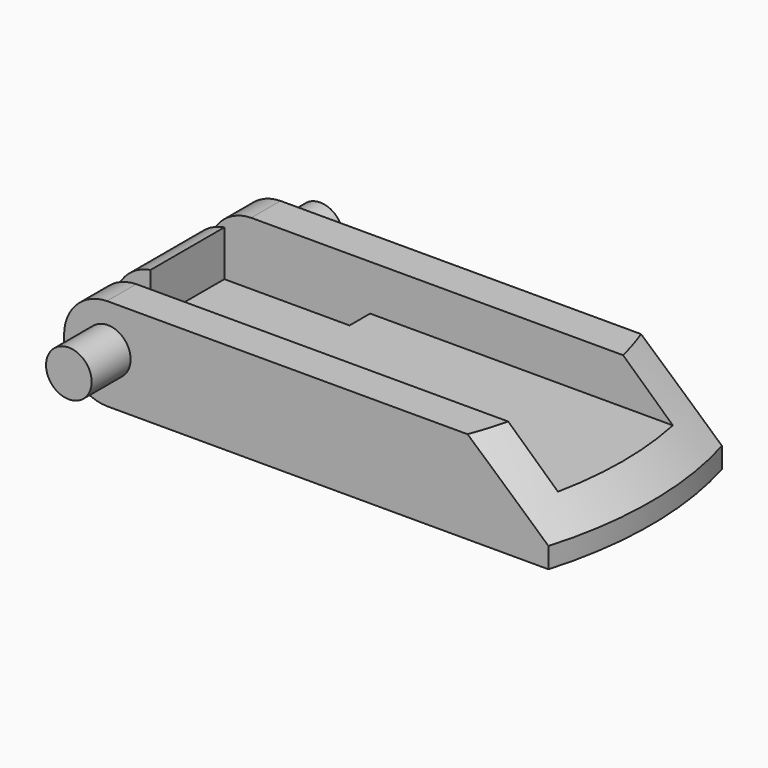
from build123d import *

# Parameters (mm, degrees)
F1_DEPTH     = 2.45
F2_W         = 1.91
F2_H         = 1.91
F2_H_2       = 4.81
F3_DEPTH     = 2.38
F4_T1_DEPTH  = 13.3148286025
F4_T3_DEPTH  = 7.6124143012
F4_T5_DEPTH  = 13.3148286025
F4_T7_DEPTH  = 16.0629874681
F4_T9_DEPTH  = 16.2148286025
F4_T14_DEPTH = 13.3148286025
F5_T2_ANGLE  = 64.9142912697
F5_T4_ANGLE  = 64.9142912697
F6_R         = 1.19
F7_DEPTH     = 2.54


# Not quite as in the source:
# - a fillet or chamfer that OpenCascade refuses, or shapes differently, is made with other operations: its cross-section is extruded or revolved along the edge and cut away or added


with BuildPart() as f1:
    # F0 (on Top) → F1 (new body)
    with BuildSketch(Plane.XY):
        Polygon((12.22, -5.655), (12.22, 5.655), (-7.02, 5.655), (-9.51, 5.655), (-13.04, 5.655), (-13.04, 3.745), (-4.6004378237, 3.745), (-4.6004378237, 2.405), (-13.04, 2.405), (-13.04, -2.405), (-4.6004378237, -2.405), (-4.6004378237, -3.745), (-13.04, -3.745), (-13.04, -5.655), (-9.51, -5.655), (-7.02, -5.655), align=None)
        with BuildLine():
            ThreePointArc((12.22, -5.655), (13.04, 0), (12.22, 5.655))
            Line((12.22, 5.655), (12.22, -5.655))
        make_face()
    extrude(amount=F1_DEPTH)

    # F2 (on face) → F3 (join)
    with BuildSketch(Plane.XY.offset(2.45)):
        with BuildLine():
            ThreePointArc((12.6846069362, 3.745), (12.4758901154, 4.705737445), (12.22, 5.655))
            Line((12.22, 5.655), (-11.13, 5.655))
            Line((-11.13, 5.655), (-11.13, 3.745))
            Line((-11.13, 3.745), (-4.6004378237, 3.745))
            Line((-4.6004378237, 3.745), (12.6846069362, 3.745))
        make_face()
        with Locations((-12.085, 4.7)):
            Rectangle(F2_W, F2_H)
        with Locations((-12.085, 0)):
            Rectangle(F2_W, F2_H_2)
        with Locations((-12.085, -4.7)):
            Rectangle(F2_W, F2_H)
        with BuildLine():
            ThreePointArc((12.22, -5.655), (12.4758901154, -4.705737445), (12.6846069362, -3.745))
            Line((12.6846069362, -3.745), (-4.6004378237, -3.745))
            Line((-4.6004378237, -3.745), (-11.13, -3.745))
            Line((-11.13, -3.745), (-11.13, -5.655))
            Line((-11.13, -5.655), (12.22, -5.655))
        make_face()
    extrude(amount=F3_DEPTH)

    # F4: fillet of radius 2.28 on 6 edges, made by hand

    # F4_s2 → F4_t1 (cut)
    with BuildSketch(Plane.XZ.offset(-1.9574143012)):
        with BuildLine():
            ThreePointArc((-10.7590343146, -0.0004), (-12.3722034611, 0.6677965389), (-13.0404, 2.2809656854))
            Line((-13.0404, 2.2809656854), (-13.2685365685, 2.2809656854))
            ThreePointArc((-13.2685365685, 2.2809656854), (-13.2681365685, 1.1404828427), (-13.2681365685, 0))
            Line((-13.2681365685, 0), (-13.04, -0.2281365685))
            ThreePointArc((-13.04, -0.2281365685), (-11.8995171573, -0.2281365685), (-10.7590343146, -0.2285365685))
            Line((-10.7590343146, -0.2285365685), (-10.7590343146, -0.0004))
        make_face()
    extrude(amount=F4_T1_DEPTH, mode=Mode.SUBTRACT)

    # F4_s4 → F4_t3 (cut)
    with BuildSketch(Plane.XZ.offset(-11.3574143012)):
        with BuildLine():
            ThreePointArc((-10.7590343146, 4.8304), (-12.3722034611, 4.1622034611), (-13.0404, 2.5490343146))
            Line((-13.0404, 2.5490343146), (-13.2685365685, 2.5490343146))
            ThreePointArc((-13.2685365685, 2.5490343146), (-13.2681365685, 3.6895171573), (-13.2681365685, 4.83))
            Line((-13.2681365685, 4.83), (-13.04, 5.0581365685))
            ThreePointArc((-13.04, 5.0581365685), (-11.8995171573, 5.0581365685), (-10.7590343146, 5.0585365685))
            Line((-10.7590343146, 5.0585365685), (-10.7590343146, 4.8304))
        make_face()
    extrude(amount=F4_T3_DEPTH, mode=Mode.SUBTRACT)

    # F4_s6 → F4_t5 (cut)
    with BuildSketch(Plane.XZ.offset(-11.3574143012)):
        with BuildLine():
            ThreePointArc((-10.7590343146, -0.0004), (-12.3722034611, 0.6677965389), (-13.0404, 2.2809656854))
            Line((-13.0404, 2.2809656854), (-13.2685365685, 2.2809656854))
            ThreePointArc((-13.2685365685, 2.2809656854), (-13.2681365685, 1.1404828427), (-13.2681365685, 0))
            Line((-13.2681365685, 0), (-13.04, -0.2281365685))
            ThreePointArc((-13.04, -0.2281365685), (-11.8995171573, -0.2281365685), (-10.7590343146, -0.2285365685))
            Line((-10.7590343146, -0.2285365685), (-10.7590343146, -0.0004))
        make_face()
    extrude(amount=F4_T5_DEPTH, mode=Mode.SUBTRACT)

    # F4_s8 → F4_t7 (cut)
    with BuildSketch(Plane.XZ.offset(-8.0314937341)):
        with BuildLine():
            ThreePointArc((-11.1300650541, 4.8303946745), (-12.4984431492, 4.0555753965), (-13.0404, 2.5794025419))
            Line((-13.0404, 2.5794025419), (-13.2685365685, 2.5794025419))
            ThreePointArc((-13.2685365685, 2.5794025419), (-13.2681365685, 3.704701271), (-13.2681365685, 4.83))
            Line((-13.2681365685, 4.83), (-13.04, 5.0581365685))
            ThreePointArc((-13.04, 5.0581365685), (-12.0850325271, 5.0581365685), (-11.1671681281, 5.0554938878))
            Line((-11.1671681281, 5.0554938878), (-11.1300650541, 4.8303946745))
        make_face()
    extrude(amount=F4_T7_DEPTH, mode=Mode.SUBTRACT)

    # F4_s10 → F4_t9 (cut)
    with BuildSketch(Plane.XZ.offset(-8.1074143012)):
        with BuildLine():
            ThreePointArc((-10.7590343146, -0.0004), (-12.3722034611, 0.6677965389), (-13.0404, 2.2809656854))
            Line((-13.0404, 2.2809656854), (-13.2685365685, 2.2809656854))
            ThreePointArc((-13.2685365685, 2.2809656854), (-13.2681365685, 1.1404828427), (-13.2681365685, 0))
            Line((-13.2681365685, 0), (-13.04, -0.2281365685))
            ThreePointArc((-13.04, -0.2281365685), (-11.8995171573, -0.2281365685), (-10.7590343146, -0.2285365685))
            Line((-10.7590343146, -0.2285365685), (-10.7590343146, -0.0004))
        make_face()
    extrude(amount=F4_T9_DEPTH, mode=Mode.SUBTRACT)


with BuildPart() as f4_tool12:
    # F4_s13 → F4_t14 (new body)
    with BuildSketch(Plane.XZ.offset(-1.9574143012)):
        with BuildLine():
            ThreePointArc((-10.7590343146, 4.8304), (-12.3722034611, 4.1622034611), (-13.0404, 2.5490343146))
            Line((-13.0404, 2.5490343146), (-13.2685365685, 2.5490343146))
            ThreePointArc((-13.2685365685, 2.5490343146), (-13.2681365685, 3.6895171573), (-13.2681365685, 4.83))
            Line((-13.2681365685, 4.83), (-13.04, 5.0581365685))
            ThreePointArc((-13.04, 5.0581365685), (-11.8995171573, 5.0581365685), (-10.7590343146, 5.0585365685))
            Line((-10.7590343146, 5.0585365685), (-10.7590343146, 4.8304))
        make_face()
    extrude(amount=F4_T14_DEPTH)

    split(bisect_by=Plane.XZ.offset(2.405), keep=Keep.TOP)


with BuildPart() as f1_1:
    add(f1.part)

    # F4_t11: cut F4_tool12
    add(f4_tool12.part, mode=Mode.SUBTRACT)

    # F5: chamfer of 4 x 3.76 on 2 edges, made by hand

    # F5_s1 → F5_t2 (revolve, cut)
    with BuildSketch(Plane(origin=(-0.7123621612, -2.0942885882, 0), x_dir=(0, 0, 1), z_dir=(-0.3220259314, -0.9467308485, 0))):
        Polygon((4.83, -9.4059274017), (1.07, -13.4059274017), (4.83, -13.4059274017), align=None)
    revolve(axis=Axis((-6.8694054878, 0, 4.83), (0, 0, 1)), revolution_arc=F5_T2_ANGLE, mode=Mode.SUBTRACT)

    # F5_s3 → F5_t4 (revolve, cut)
    with BuildSketch(Plane(origin=(-3.5700040609, -3.4320367849, 0), x_dir=(0, 0, 1), z_dir=(-0.7208995903, -0.6930395232, 0))):
        Polygon((4.83, -11.148635984), (1.07, -15.148635984), (4.83, -15.148635984), align=None)
    revolve(axis=Axis((-6.8694054878, 0, 4.83), (0, 0, 1)), revolution_arc=F5_T4_ANGLE, mode=Mode.SUBTRACT)

    # F6 (on face) → F7 (join)
    with BuildSketch(Plane.XZ.offset(5.655)):
        with Locations((-10.76, 2.55)):
            Circle(F6_R)
    extrude(amount=F7_DEPTH)

    # F8: F1 across plane


with BuildPart() as f1_2:
    add(f1_1.part)
    add(f1_1.part.mirror(Plane.XZ))


solid = f1_2.part
